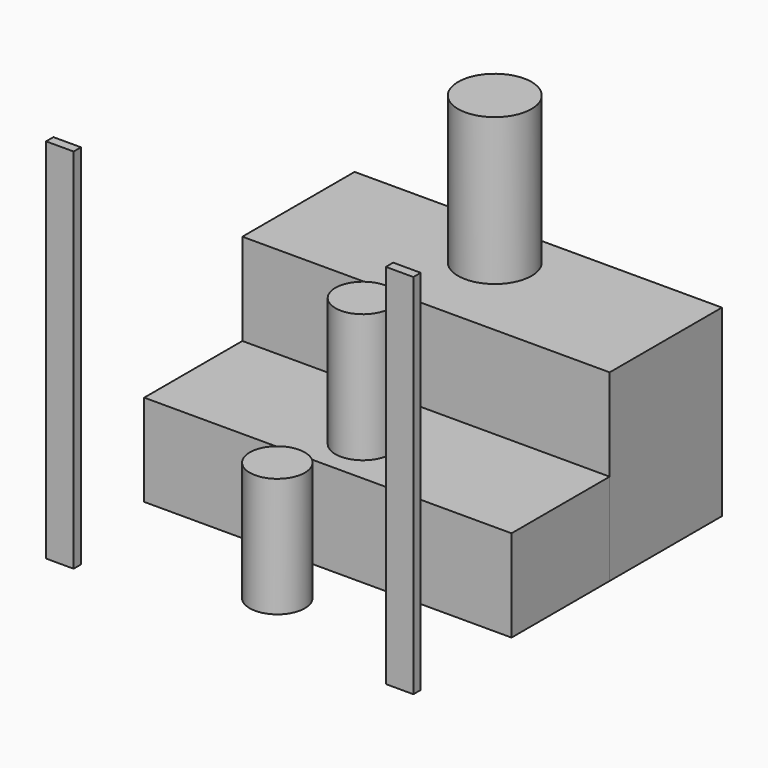
from build123d import *

# Parameters (mm, degrees)
F5_W      = 19.05
F5_H      = 254
F6_DEPTH  = 6.35
F7_W      = 254
F7_H      = 84.836
F8_DEPTH  = 63.5
F7_H_2    = 97.028
F9_DEPTH  = 127
F10_R     = 19.05
F11_DEPTH = 82.55
F12_R     = 19.05
F13_DEPTH = 88.9
F14_R     = 25.4
F15_DEPTH = 101.6


# Not quite as in the source:
# - the program builds the solid bodies; features that only make, move or delete a surface that nothing else refers to are left out


with BuildPart() as f6:
    # F5 (on Front) → F6 (new body)
    with BuildSketch(Plane.XZ):
        with Locations((-244.475, 127)):
            Rectangle(F5_W, F5_H)
    extrude(amount=-F6_DEPTH)


with BuildPart() as f6b:
    # F5 (on Front) → F6, piece 2 (new body)
    with BuildSketch(Plane.XZ):
        with Locations((-9.525, 127)):
            Rectangle(F5_W, F5_H)
    extrude(amount=-F6_DEPTH)


with BuildPart() as f8:
    # F7 (on face) → F8 (new body)
    with BuildSketch(Plane(origin=(0, 0, 0), x_dir=(1, 0, 0), z_dir=(0, 0, -1))):
        with Locations((-127, -127.254)):
            Rectangle(F7_W, F7_H)
    extrude(amount=-F8_DEPTH)

    # F12 (on face) → F13 (join)
    with BuildSketch(Plane.XY.offset(63.5)):
        with Locations((-127.8826892376, 116.2502095103)):
            Circle(F12_R)
    extrude(amount=F13_DEPTH)


with BuildPart() as f9:
    # F7 (on face) → F9 (new body)
    with BuildSketch(Plane(origin=(0, 0, 0), x_dir=(1, 0, 0), z_dir=(0, 0, -1))):
        with Locations((-127, -218.186)):
            Rectangle(F7_W, F7_H_2)
    extrude(amount=-F9_DEPTH)

    # F14 (on face) → F15 (join)
    with BuildSketch(Plane.XY.offset(127)):
        with Locations((-128.804281354, 231.3739955425)):
            Circle(F14_R)
    extrude(amount=F15_DEPTH)


with BuildPart() as f11:
    # F10 (on face) → F11 (new body)
    with BuildSketch(Plane(origin=(0, 0, 0), x_dir=(1, 0, 0), z_dir=(0, 0, -1))):
        with Locations((-127.6017278433, -41.8717749417)):
            Circle(F10_R)
    extrude(amount=-F11_DEPTH)


solid = Compound([f6.part, f6b.part, f8.part, f9.part, f11.part])
